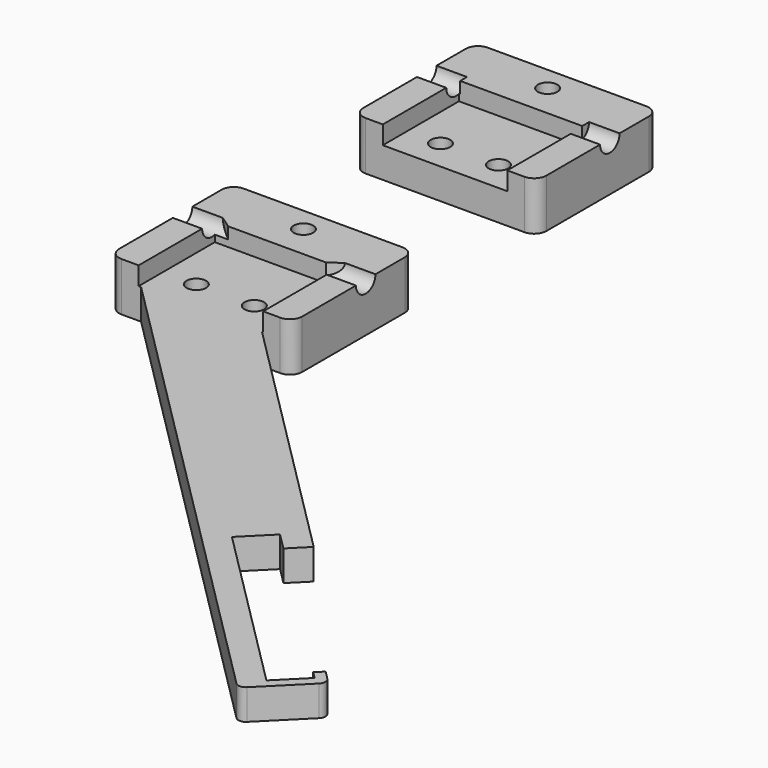
from build123d import *

# Parameters (mm, degrees)
F1_DEPTH  = 8
F2_W      = 20.4
F2_H      = 15.6
F3_DEPTH  = 3
F4_R      = 2
F5_DEPTH  = 5
F6_R      = 2
F7_DEPTH  = 5
F8_R      = 1.6
F9_DEPTH  = 5.001
F10_R     = 1.6
F11_DEPTH = 8.001
F14_DEPTH = 3
F16_DEPTH = 5
F17_SIZE2 = 1.399415
F17_SIZE  = 1.999
F18_SIZE2 = 1.399415
F18_SIZE  = 1.999


# Not quite as in the source:
# - a fillet or chamfer is up to 0.001 mm smaller than in the source, because OpenCascade refuses the exact size


with BuildPart() as f1:
    # F0 (on Top) → F1 (new body)
    with BuildSketch(Plane.XY):
        with BuildLine():
            Line((13, 11.9621065401), (-13, 11.9621065401))
            ThreePointArc((-13, 11.9621065401), (-14.4142135624, 11.3763201025), (-15, 9.9621065401))
            Line((-15, 9.9621065401), (-15, -11.0378934599))
            ThreePointArc((-15, -11.0378934599), (-14.4142135624, -12.4521070223), (-13, -13.0378934599))
            Line((-13, -13.0378934599), (13, -13.0378934599))
            ThreePointArc((13, -13.0378934599), (14.4142135624, -12.4521070223), (15, -11.0378934599))
            Line((15, -11.0378934599), (15, 9.9621065401))
            ThreePointArc((15, 9.9621065401), (14.4142135624, 11.3763201025), (13, 11.9621065401))
        make_face()
    extrude(amount=F1_DEPTH)

    # F2 (on face) → F3 (cut)
    with BuildSketch(Plane.XY.offset(8)):
        with Locations((0, -5.2378934599)):
            Rectangle(F2_W, F2_H)
    extrude(amount=-F3_DEPTH, mode=Mode.SUBTRACT)

    # F4 (on face) → F5 (cut)
    with BuildSketch(Plane.YZ.offset(15)):
        with Locations((1.9621065401, 8)):
            Circle(F4_R)
    extrude(amount=-F5_DEPTH, mode=Mode.SUBTRACT)

    # F6 (on face) → F7 (cut)
    with BuildSketch(Plane(origin=(-15, 0, 0), x_dir=(0, -1, 0), z_dir=(-1, 0, 0))):
        with Locations((-1.9621065401, 8)):
            Circle(F6_R)
    extrude(amount=-F7_DEPTH, mode=Mode.SUBTRACT)

    # F8 (on face) → F9 (cut, through all)
    with BuildSketch(Plane.XY.offset(5)):
        with Locations((-4.75, -8.0378934599)):
            Circle(F8_R)
        with Locations((4.75, -8.0378934599)):
            Circle(F8_R)
    extrude(amount=-F9_DEPTH, mode=Mode.SUBTRACT)

    # F10 (on face) → F11 (cut, through all)
    with BuildSketch(Plane.XY.offset(8)):
        with Locations((0, 7.9621065401)):
            Circle(F10_R)
    extrude(amount=-F11_DEPTH, mode=Mode.SUBTRACT)


with BuildPart() as f12_1:
    # F12: copy of F1
    add(f1.part.moved(Location((0, -50, 0))))

    # F13 (on face) → F14 (cut)
    with BuildSketch(Plane(origin=(0, 0, 0), x_dir=(1, 0, 0), z_dir=(0, 0, -1))):
        Polygon((-3.1622867597, 55.2878934599), (-1.5745735195, 58.0378934599), (-3.1622867597, 60.7878934599), (-6.3377132403, 60.7878934599), (-7.9254264805, 58.0378934599), (-6.3377132403, 55.2878934599), align=None)
        Polygon((6.3377132403, 55.2878934599), (7.9254264805, 58.0378934599), (6.3377132403, 60.7878934599), (3.1622867597, 60.7878934599), (1.5745735195, 58.0378934599), (3.1622867597, 55.2878934599), align=None)
        Polygon((-1.5877132403, 39.2878934599), (1.5877132403, 39.2878934599), (3.1754264805, 42.0378934599), (1.5877132403, 44.7878934599), (-1.5877132403, 44.7878934599), (-3.1754264805, 42.0378934599), align=None)
    extrude(amount=-F14_DEPTH, mode=Mode.SUBTRACT)

    # F15 (on face) → F16 (join)
    with BuildSketch(Plane(origin=(0, 0, 0), x_dir=(1, 0, 0), z_dir=(0, 0, -1))):
        with BuildLine():
            Line((-9.7989898732, 63.0378934599), (10, 63.0378934599))
            Line((10, 63.0378934599), (52.4264068712, 105.4643003311))
            Line((52.4264068712, 105.4643003311), (49.6686904246, 108.2220167777))
            Line((49.6686904246, 108.2220167777), (46.9109739779, 105.4643003311))
            Line((46.9109739779, 105.4643003311), (42.5269119346, 109.8483623745))
            Line((42.5269119346, 109.8483623745), (70.811183182, 138.1326336219))
            Line((70.811183182, 138.1326336219), (75.1952452254, 133.7485715786))
            Line((75.1952452254, 133.7485715786), (74.0638743755, 132.6172007287))
            Line((74.0638743755, 132.6172007287), (75.1952452254, 131.4858298788))
            Line((75.1952452254, 131.4858298788), (76.6094587878, 132.9000434412))
            ThreePointArc((76.6094587878, 132.9000434412), (76.9609306503, 133.7485715786), (76.6094587878, 134.597099716))
            Line((76.6094587878, 134.597099716), (70.0333657227, 141.173192781))
            ThreePointArc((70.0333657227, 141.173192781), (69.1848375853, 141.5246646436), (68.3363094479, 141.173192781))
            Line((68.3363094479, 141.173192781), (-9.7989898732, 63.0378934599))
        make_face()
    extrude(amount=-F16_DEPTH)

    # F17 (size 2 and 1.4004150764 in the source; OpenCascade refuses exactly that, so slightly less here)
    f17_edges = [f12_1.edges().sort_by_distance(p)[0] for p in [
        (-10, -47.437893, 7.046061),
    ]]
    f17_side = f12_1.faces().sort_by_distance((0, -47.437893, 6.493105))[0]
    chamfer(f17_edges, length=F17_SIZE, length2=F17_SIZE2, reference=f17_side)

    # F18 (size 2 and 1.4004150764 in the source; OpenCascade refuses exactly that, so slightly less here)
    f18_edges = [f12_1.edges().sort_by_distance(p)[0] for p in [
        (10, -47.437893, 7.046061),
    ]]
    f18_side = f12_1.faces().sort_by_distance((0.60623, -47.437893, 6.45586))[0]
    chamfer(f18_edges, length=F18_SIZE, length2=F18_SIZE2, reference=f18_side)


solid = Compound([f1.part, f12_1.part])
